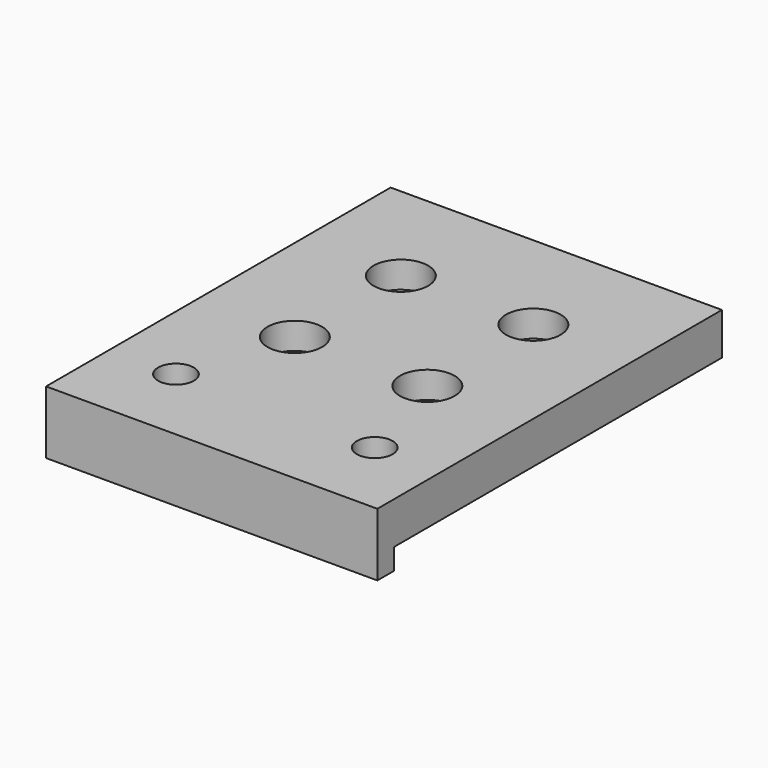
from build123d import *

# Parameters (mm, degrees)
F0_W           = 50
F0_H           = 65
F1_DEPTH       = 9.525
F2_W           = 50
F2_H           = 61.825
F3_DEPTH       = 3.175
F5_D           = 4.4
F5_CBORE_D     = 8.25
F5_CBORE_DEPTH = 4
F7_D           = 5.4


# Not quite as in the source:
# - a length typed as a fraction of an inch, garbled in the dataset ("3 / 203.2 mm" for 3/8 in), is restored


with BuildPart() as f1:
    # F0 (on Top) → F1 (new body)
    with BuildSketch(Plane.XY):
        Rectangle(F0_W, F0_H)
    extrude(amount=F1_DEPTH)

    # F2 (on face) → F3 (cut)
    with BuildSketch(Plane(origin=(0, 0, 0), x_dir=(1, 0, 0), z_dir=(0, 0, -1))):
        with Locations((0, -1.5875)):
            Rectangle(F2_W, F2_H)
    extrude(amount=-F3_DEPTH, mode=Mode.SUBTRACT)

    # F5 (through all)
    with Locations(Plane.XY.offset(9.525)):
        with Locations((-10, 15.675), (10, 15.675), (10, -4.325), (-10, -4.325)):
            CounterBoreHole(F5_D / 2, F5_CBORE_D / 2, F5_CBORE_DEPTH)

    # F7 (through all)
    with Locations(Plane.XY.offset(9.525)):
        with Locations((-15, -20.5), (15, -20.5)):
            Hole(F7_D / 2)


solid = f1.part
